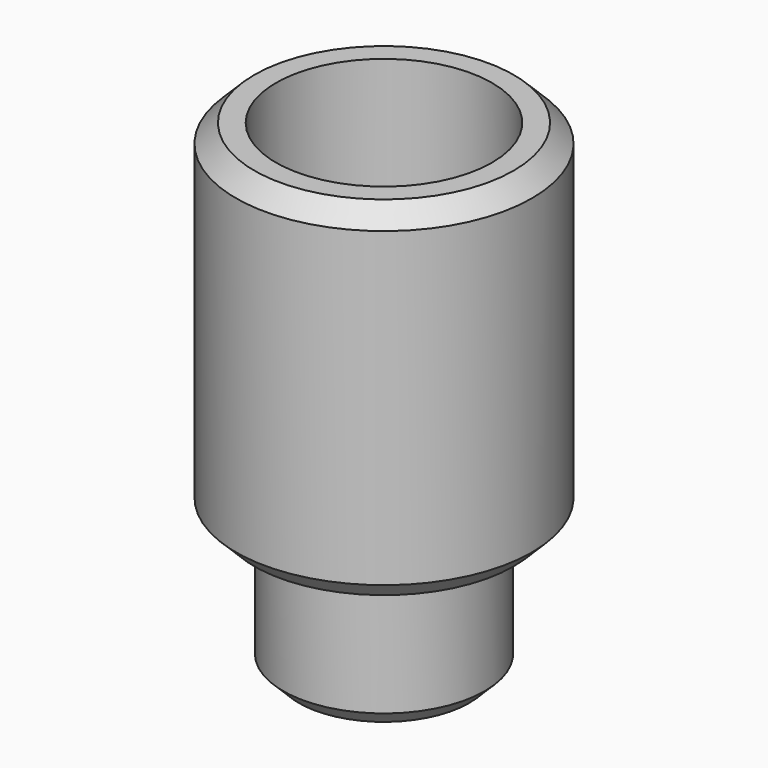
from build123d import *

# Parameters (mm, degrees)
F0_R     = 11
F1_DEPTH = 15
F2_R     = 16.15
F3_DEPTH = 38
F4_R     = 9.3
F5_DEPTH = 53.001
F7_R     = 11.7844294456
F8_DEPTH = 25


# Not quite as in the source:
# - a fillet or chamfer that OpenCascade refuses, or shapes differently, is made with other operations: its cross-section is extruded or revolved along the edge and cut away or added


with BuildPart() as f1:
    # F0 (on Top) → F1 (new body)
    with BuildSketch(Plane.XY):
        Circle(F0_R)
    extrude(amount=F1_DEPTH)

    # F2 (on face) → F3 (join)
    with BuildSketch(Plane.XY.offset(15)):
        Circle(F2_R)
    extrude(amount=F3_DEPTH)

    # F4 (on face) → F5 (cut, through all)
    with BuildSketch(Plane(origin=(0, 0, 0), x_dir=(1, 0, 0), z_dir=(0, 0, -1))):
        Circle(F4_R)
    extrude(amount=-F5_DEPTH, mode=Mode.SUBTRACT)

    # F7 (on offset) → F8 (cut)
    with BuildSketch(Plane.XY.offset(55)):
        Circle(F7_R)
    extrude(amount=-F8_DEPTH, mode=Mode.SUBTRACT)

    # F9: chamfer of 2 on 3 edges, made by hand

    # F9_s1 → F9_t2 (revolve, cut)
    with BuildSketch(Plane.XZ):
        Polygon((16.15, 51), (14.15, 53), (16.15, 53), align=None)
    revolve(axis=Axis((0, 0, 53), (0, 0, 1)), mode=Mode.SUBTRACT)

    # F9_s3 → F9_t4 (revolve, cut)
    with BuildSketch(Plane.XZ):
        Polygon((11, 2), (9, 0), (11, 0), align=None)
    revolve(axis=Axis((0, 0, 0), (0, 0, 1)), mode=Mode.SUBTRACT)

    # F9_s5 → F9_t6 (revolve, cut)
    with BuildSketch(Plane.XZ):
        Polygon((16.15, 17), (14.15, 15), (16.15, 15), align=None)
    revolve(axis=Axis((0, 0, 15), (0, 0, 1)), mode=Mode.SUBTRACT)


solid = f1.part
